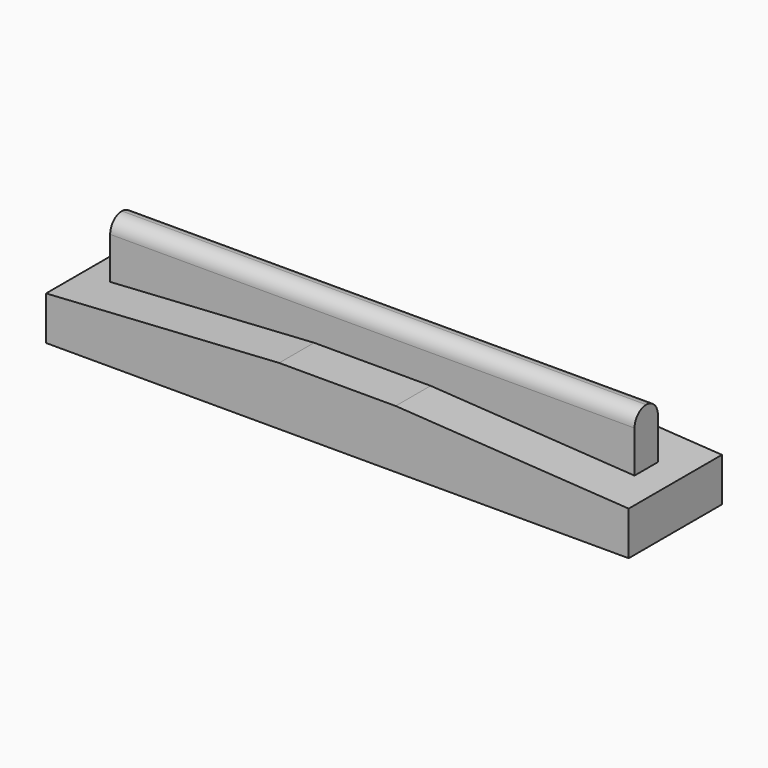
from build123d import *

# Parameters (mm, degrees)
F0_W        = 63.5
F0_H        = 12.7
F0_W_2      = 57.15
F0_H_2      = 3.175
F1_DEPTH    = 1.5875
F2_DEPTH    = 1.5875
F3_DEPTH    = 6.35
F4_R        = 1.58749
F5_T1_DEPTH = 144.7704872523
F6_DEPTH    = 3.175


# Not quite as in the source:
# - a fillet or chamfer that OpenCascade refuses, or shapes differently, is made with other operations: its cross-section is extruded or revolved along the edge and cut away or added
# - a fillet or chamfer is up to 0.001 mm smaller than in the source, because OpenCascade refuses the exact size


with BuildPart() as f1:
    # F0 (on Top) → F1 (new body, symmetric)
    with BuildSketch(Plane.XY):
        Rectangle(F0_W, F0_H)
        Rectangle(F0_W_2, F0_H_2, mode=Mode.SUBTRACT)
    extrude(amount=F1_DEPTH, both=True)

    # F0 (on Top) → F2 (join)
    with BuildSketch(Plane.XY):
        Rectangle(F0_W_2, F0_H_2)
    extrude(amount=-F2_DEPTH)

    # F5: chamfer of 25.4 x 1.5875 on 2 edges, made by hand

    # F5_s2 → F5_t1 (cut)
    with BuildSketch(Plane.XZ.offset(-72.3852436262)):
        Polygon((-6.35, 1.5875), (-31.75, 0), (-31.75, 1.5875), align=None)
        Polygon((31.75, 0), (6.35, 1.5875), (31.75, 1.5875), align=None)
    extrude(amount=F5_T1_DEPTH, mode=Mode.SUBTRACT)

    # F6 (add): a face of the model
    f6_faces = [f1.faces().sort_by_distance(p)[0] for p in [
        (0, 0, -1.5875),
    ]]
    extrude(f6_faces, amount=F6_DEPTH)


with BuildPart() as f3:
    # F0 (on Top) → F3 (new body)
    with BuildSketch(Plane.XY):
        Rectangle(F0_W_2, F0_H_2)
    extrude(amount=F3_DEPTH)

    # F4 (radius 1.5875 in the source; OpenCascade refuses exactly that, so slightly less here)
    f4_edges = [f3.edges().sort_by_distance(p)[0] for p in [
        (0, -1.5875, 6.35),
        (0, 1.5875, 6.35),
    ]]
    fillet(f4_edges, radius=F4_R)


solid = Compound([f1.part, f3.part])
